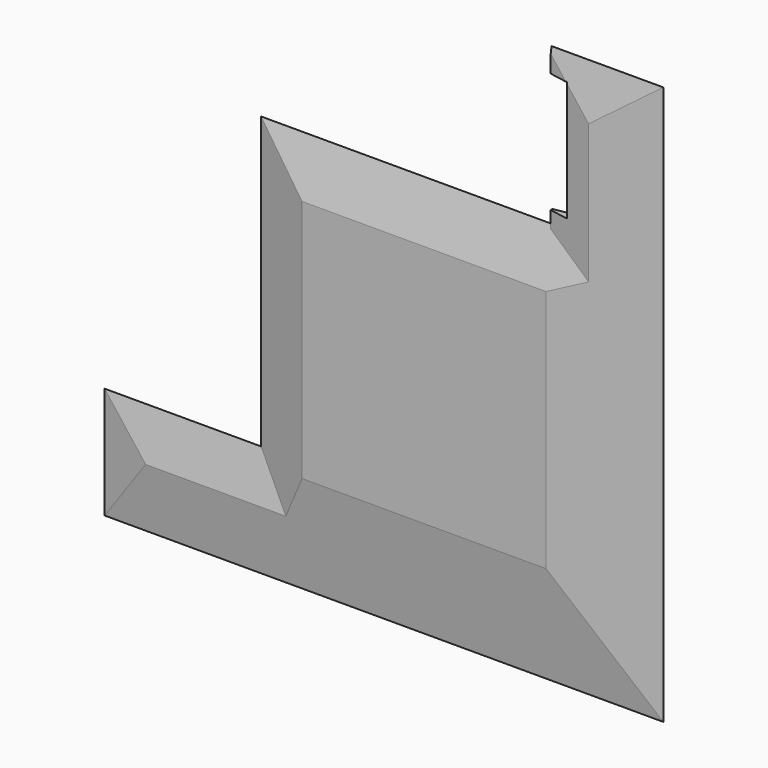
from build123d import *

# Parameters (mm, degrees)
F1_DEPTH    = 50
F3_SIZE2    = 141.7820454904
F3_SIZE     = 25
F4_SIZE2    = 24.99999
F4_SIZE     = 189.893843
F5_SIZE2    = 141.782035
F5_SIZE     = 24.99999
F5_2_SIZE2  = 141.782035
F5_2_SIZE   = 24.99999
F6_T1_DEPTH = 477.1700191754
F7_T1_DEPTH = 506.6441108429
F8_SIZE2    = 25
F8_SIZE     = 93.3012701892
F8_2_SIZE2  = 24.99999
F8_2_SIZE   = 93.30126
F10_DEPTH   = 25


# Not quite as in the source:
# - a fillet or chamfer that OpenCascade refuses, or shapes differently, is made with other operations: its cross-section is extruded or revolved along the edge and cut away or added
# - a fillet or chamfer is up to 0.001 mm smaller than in the source, because OpenCascade refuses the exact size


with BuildPart() as f1:
    # F0 (on Front) → F1 (new body)
    with BuildSketch(Plane.XZ):
        Polygon((0, 200), (0, 0), (1000, 0), (1000, 1000), (800, 1000), (800, 720), (280, 720), (280, 200), align=None)
    extrude(amount=F1_DEPTH)


with BuildPart() as f1_1:
    # F2: moved
    add(f1.part.moved(Location((1592, 0, 0))))

    # F3
    f3_edges = [f1_1.edges().sort_by_distance(p)[0] for p in [
        (2592, 0, 500),
        (2092, 0, 0),
    ]]
    chamfer(f3_edges, length=F3_SIZE, length2=F3_SIZE2)

    # F4 (size 189.8938528181 and 25 in the source; OpenCascade refuses exactly that, so slightly less here)
    f4_edges = [f1_1.edges().sort_by_distance(p)[0] for p in [
        (2092, -50, 0),
        (2592, -50, 500),
    ]]
    f4_side = f1_1.faces().sort_by_distance((2210.680203, -50, 381.319797))[0]
    chamfer(f4_edges, length=F4_SIZE, length2=F4_SIZE2, reference=f4_side)

    # F5 (size 25 and 141.7820454904 in the source; OpenCascade refuses exactly that, so slightly less here)
    f5_edges = [f1_1.edges().sort_by_distance(p)[0] for p in [
        (2421.108977, 0, 1000),
        (2397.053079, -50, 1000),
    ]]
    f5_side = f1_1.faces().sort_by_distance((2461.151755, -23.287804, 1000))[0]
    chamfer(f5_edges, length=F5_SIZE, length2=F5_SIZE2, reference=f5_side)

    # F5#2 (size 25 and 141.7820454904 in the source; OpenCascade refuses exactly that, so slightly less here)
    f5_2_edges = [f1_1.edges().sort_by_distance(p)[0] for p in [
        (1592, 0, 170.891023),
        (1592, -50, 194.946922),
    ]]
    f5_2_side = f1_1.faces().sort_by_distance((1592, -23.287804, 130.848245))[0]
    chamfer(f5_2_edges, length=F5_2_SIZE, length2=F5_2_SIZE2, reference=f5_2_side)

    # F6: chamfer of 23 x 130.4394818512 on 2 edges, made by hand

    # F6_s2 → F6_t1 (cut)
    with BuildSketch(Plane.XY.offset(720)):
        Polygon((2522.4394818512, -50), (2392, -27), (2392, -50), align=None)
        Polygon((2392, -23), (2522.4394818512, 0), (2392, 0), align=None)
    extrude(amount=F6_T1_DEPTH, mode=Mode.SUBTRACT)

    # F7: chamfer of 25 x 141.7820454904 on 2 edges, made by hand

    # F7_s2 → F7_t1 (cut)
    with BuildSketch(Plane.YZ.offset(1365.3558891571)):
        Polygon((-25, 200), (0, 58.2179545096), (0, 200), align=None)
        Polygon((-50, 58.2179545096), (-25, 200), (-50, 200), align=None)
    extrude(amount=F7_T1_DEPTH, mode=Mode.SUBTRACT)

    # F8
    f8_edges = [f1_1.edges().sort_by_distance(p)[0] for p in [
        (1872, 0, 430.891023),
        (2161.108977, 0, 720),
    ]]
    f8_side = f1_1.faces().sort_by_distance((2161.108977, 0, 430.891023))[0]
    chamfer(f8_edges, length=F8_SIZE, length2=F8_SIZE2, reference=f8_side)

    # F8#2 (size 93.3012701892 and 25 in the source; OpenCascade refuses exactly that, so slightly less here)
    f8_2_edges = [f1_1.edges().sort_by_distance(p)[0] for p in [
        (1872, -50, 454.946922),
        (2137.053079, -50, 720),
    ]]
    f8_2_side = f1_1.faces().sort_by_distance((2137.053079, -50, 454.946921))[0]
    chamfer(f8_2_edges, length=F8_2_SIZE, length2=F8_2_SIZE2, reference=f8_2_side)

    # F9 (on face) → F10 (cut)
    with BuildSketch(Plane(origin=(76.0608571883, -431.3625565565, 0), x_dir=(-0.984807753, -0.1736481777, 0), z_dir=(-0.1736481777, 0.984807753, 0))):
        Polygon((-2346.6920852661, 742.4287796021), (-2347.2633361816, 957.3464989662), (-2383.4601961924, 957.3464989662), (-2383.4601961924, 742.4287796021), align=None)
    extrude(amount=-F10_DEPTH, mode=Mode.SUBTRACT)


solid = f1_1.part
